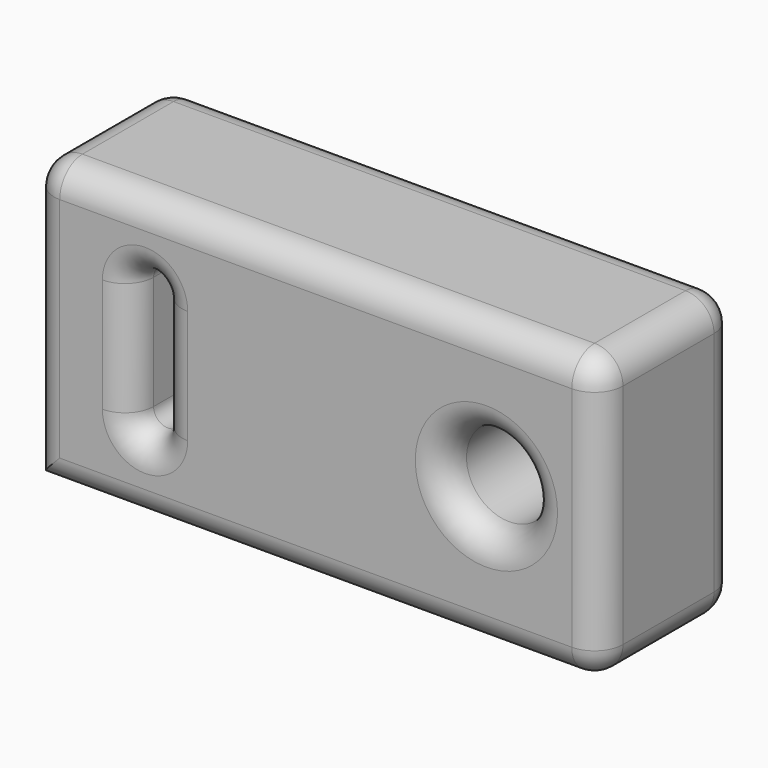
from build123d import *

# Parameters (mm, degrees)
F0_W         = 254
F0_H         = 127
F1_DEPTH     = 76.2
F2_R         = 19.05
F3_DEPTH     = 76.201
F5_DEPTH     = 76.201
F6_R         = 12.7
F7_T1_DEPTH  = 228.6
F7_T3_DEPTH  = 50.8
F7_T5_DEPTH  = 101.6
F7_T7_DEPTH  = 273.05
F7_T9_DEPTH  = 146.05
F7_T11_DEPTH = 50.8
F7_S15_W     = 12.7
F7_S15_H     = 12.7
F7_T16_DEPTH = 12.7
F7_S21_W     = 12.7
F7_S21_H     = 12.7
F7_T22_DEPTH = 12.7
F7_S27_W     = 12.7
F7_S27_H     = 12.7
F7_T28_DEPTH = 12.7
F7_S33_W     = 12.7
F7_S33_H     = 12.7
F7_T34_DEPTH = 12.7
F7_S39_W     = 12.7
F7_S39_H     = 12.7
F7_T40_DEPTH = 12.7
F7_S45_W     = 12.7
F7_S45_H     = 12.7
F7_T46_DEPTH = 12.7
F7_T50_ANGLE = 180
F7_T52_ANGLE = 180


# Not quite as in the source:
# - a fillet or chamfer that OpenCascade refuses, or shapes differently, is made with other operations: its cross-section is extruded or revolved along the edge and cut away or added


with BuildPart() as f1:
    # F0 (on Front) → F1 (new body)
    with BuildSketch(Plane.XZ):
        with Locations((127, 63.5)):
            Rectangle(F0_W, F0_H)
    extrude(amount=F1_DEPTH)

    # F2 (on face) → F3 (cut, through all)
    with BuildSketch(Plane.XZ.offset(76.2)):
        with Locations((203.2, 63.5)):
            Circle(F2_R)
    extrude(amount=-F3_DEPTH, mode=Mode.SUBTRACT)

    # F4 (on face) → F5 (cut, through all)
    with BuildSketch(Plane.XZ.offset(76.2)):
        with BuildLine():
            Line((57.15, 38.1), (57.15, 88.9))
            ThreePointArc((57.15, 88.9), (50.8, 95.25), (44.45, 88.9))
            Line((44.45, 88.9), (44.45, 38.1))
            ThreePointArc((44.45, 38.1), (50.8, 31.75), (57.15, 38.1))
        make_face()
    extrude(amount=-F5_DEPTH, mode=Mode.SUBTRACT)

    # F6
    f6_edges = [f1.edges().sort_by_distance(p)[0] for p in [
        (0, -76.2, 63.5),
        (127, -76.2, 127),
        (127, -76.2, 0),
        (254, -76.2, 63.5),
        (57.15, -76.2, 63.5),
        (50.8, -76.2, 95.25),
        (44.45, -76.2, 63.5),
        (50.8, -76.2, 31.75),
        (184.15, -76.2, 63.5),
    ]]
    fillet(f6_edges, radius=F6_R)

    # F7: fillet of radius 12.7 on 12 edges, made by hand

    # F7_s2 → F7_t1 (cut)
    with BuildSketch(Plane.YZ.offset(12.7)):
        with BuildLine():
            ThreePointArc((-12.7, 127), (-3.7197438789, 123.2802561211), (0, 114.3))
            Line((0, 114.3), (0, 127))
            Line((0, 127), (-12.7, 127))
        make_face()
    extrude(amount=F7_T1_DEPTH, mode=Mode.SUBTRACT)

    # F7_s4 → F7_t3 (cut)
    with BuildSketch(Plane.XZ.offset(12.7)):
        with BuildLine():
            ThreePointArc((0, 114.3), (3.7197438789, 123.2802561211), (12.7, 127))
            Line((12.7, 127), (0, 127))
            Line((0, 127), (0, 114.3))
        make_face()
        with BuildLine():
            ThreePointArc((241.3, 127), (250.2802561211, 123.2802561211), (254, 114.3))
            Line((254, 114.3), (254, 127))
            Line((254, 127), (241.3, 127))
        make_face()
        with BuildLine():
            ThreePointArc((241.3, 0), (250.2802561211, 3.7197438789), (254, 12.7))
            Line((254, 12.7), (254, 0))
            Line((254, 0), (241.3, 0))
        make_face()
    extrude(amount=F7_T3_DEPTH, mode=Mode.SUBTRACT)

    # F7_s6 → F7_t5 (cut)
    with BuildSketch(Plane.XY.offset(12.7)):
        with BuildLine():
            ThreePointArc((241.3, 0), (250.2802561211, -3.7197438789), (254, -12.7))
            Line((254, -12.7), (254, 0))
            Line((254, 0), (241.3, 0))
        make_face()
    extrude(amount=F7_T5_DEPTH, mode=Mode.SUBTRACT)

    # F7_s8 → F7_t7 (cut)
    with BuildSketch(Plane.YZ.offset(-31.75)):
        with BuildLine():
            ThreePointArc((0, 12.7), (-3.7197438789, 3.7197438789), (-12.7, 0))
            Line((-12.7, 0), (0, 0))
            Line((0, 0), (0, 12.7))
        make_face()
    extrude(amount=F7_T7_DEPTH, mode=Mode.SUBTRACT)

    # F7_s10 → F7_t9 (cut)
    with BuildSketch(Plane.XY.offset(-31.75)):
        with BuildLine():
            ThreePointArc((0, -12.7), (3.7197438789, -3.7197438789), (12.7, 0))
            Line((12.7, 0), (0, 0))
            Line((0, 0), (0, -12.7))
        make_face()
    extrude(amount=F7_T9_DEPTH, mode=Mode.SUBTRACT)

    # F7_s12 → F7_t11 (cut)
    with BuildSketch(Plane.XY.offset(38.1)):
        with BuildLine():
            ThreePointArc((31.75, 0), (40.7302561211, -3.7197438789), (44.45, -12.7))
            Line((44.45, -12.7), (44.45, 0))
            Line((44.45, 0), (31.75, 0))
        make_face()
        with BuildLine():
            ThreePointArc((69.85, 0), (60.8697438789, -3.7197438789), (57.15, -12.7))
            Line((57.15, -12.7), (57.15, 0))
            Line((57.15, 0), (69.85, 0))
        make_face()
    extrude(amount=F7_T11_DEPTH, mode=Mode.SUBTRACT)


with BuildPart() as f7_tool14:
    # F7_s15 → F7_t16 (new body)
    with BuildSketch(Plane.XY.offset(12.7)):
        with Locations((247.65, -69.85)):
            Rectangle(F7_S15_W, F7_S15_H)
    extrude(amount=-F7_T16_DEPTH)

    # F7_s17 → F7_t18 (revolve, cut)
    with BuildSketch(Plane(origin=(241.3, -63.5, 12.7), x_dir=(-0.7071067812, 0.7071067812, 0), z_dir=(-0.7071067812, -0.7071067812, 0))):
        with BuildLine():
            ThreePointArc((0, -12.7), (12.7, 0), (0, 12.7))
            Line((0, 12.7), (0, -12.7))
        make_face()
    revolve(axis=Axis((241.3, -63.5, 12.7), (0, 0, -1)), mode=Mode.SUBTRACT)


with BuildPart() as f1_1:
    add(f1.part)

    # F7_t13: cut F7_tool14
    add(f7_tool14.part, mode=Mode.SUBTRACT)


with BuildPart() as f7_tool20:
    # F7_s21 → F7_t22 (new body)
    with BuildSketch(Plane.XY.offset(114.3)):
        with Locations((247.65, -69.85)):
            Rectangle(F7_S21_W, F7_S21_H)
    extrude(amount=F7_T22_DEPTH)

    # F7_s23 → F7_t24 (revolve, cut)
    with BuildSketch(Plane(origin=(241.3, -63.5, 114.3), x_dir=(-0.7071067812, 0.7071067812, 0), z_dir=(0.7071067812, 0.7071067812, 0))):
        with BuildLine():
            ThreePointArc((0, -12.7), (12.7, 0), (0, 12.7))
            Line((0, 12.7), (0, -12.7))
        make_face()
    revolve(axis=Axis((241.3, -63.5, 114.3), (0, 0, 1)), mode=Mode.SUBTRACT)


with BuildPart() as f1_2:
    add(f1_1.part)

    # F7_t19: cut F7_tool20
    add(f7_tool20.part, mode=Mode.SUBTRACT)


with BuildPart() as f7_tool26:
    # F7_s27 → F7_t28 (new body)
    with BuildSketch(Plane.YZ.offset(12.7)):
        with Locations((-69.85, 120.65)):
            Rectangle(F7_S27_W, F7_S27_H)
    extrude(amount=-F7_T28_DEPTH)

    # F7_s29 → F7_t30 (revolve, cut)
    with BuildSketch(Plane(origin=(12.7, -63.5, 114.3), x_dir=(0, 0.7071067812, -0.7071067812), z_dir=(0, 0.7071067812, 0.7071067812))):
        with BuildLine():
            ThreePointArc((0, -12.7), (12.7, 0), (0, 12.7))
            Line((0, 12.7), (0, -12.7))
        make_face()
    revolve(axis=Axis((12.7, -63.5, 114.3), (-1, 0, 0)), mode=Mode.SUBTRACT)


with BuildPart() as f1_3:
    add(f1_2.part)

    # F7_t25: cut F7_tool26
    add(f7_tool26.part, mode=Mode.SUBTRACT)


with BuildPart() as f7_tool32:
    # F7_s33 → F7_t34 (new body)
    with BuildSketch(Plane.XY.offset(114.3)):
        with Locations((247.65, -6.35)):
            Rectangle(F7_S33_W, F7_S33_H)
    extrude(amount=F7_T34_DEPTH)

    # F7_s35 → F7_t36 (revolve, cut)
    with BuildSketch(Plane(origin=(241.3, -12.7, 114.3), x_dir=(-0.7071067812, -0.7071067812, 0), z_dir=(-0.7071067812, 0.7071067812, 0))):
        with BuildLine():
            ThreePointArc((0, -12.7), (12.7, 0), (0, 12.7))
            Line((0, 12.7), (0, -12.7))
        make_face()
    revolve(axis=Axis((241.3, -12.7, 114.3), (0, 0, 1)), mode=Mode.SUBTRACT)


with BuildPart() as f1_4:
    add(f1_3.part)

    # F7_t31: cut F7_tool32
    add(f7_tool32.part, mode=Mode.SUBTRACT)


with BuildPart() as f7_tool38:
    # F7_s39 → F7_t40 (new body)
    with BuildSketch(Plane.YZ.offset(12.7)):
        with Locations((-6.35, 120.65)):
            Rectangle(F7_S39_W, F7_S39_H)
    extrude(amount=-F7_T40_DEPTH)

    # F7_s41 → F7_t42 (revolve, cut)
    with BuildSketch(Plane(origin=(12.7, -12.7, 114.3), x_dir=(0, -0.7071067812, -0.7071067812), z_dir=(0, 0.7071067812, -0.7071067812))):
        with BuildLine():
            ThreePointArc((0, -12.7), (12.7, 0), (0, 12.7))
            Line((0, 12.7), (0, -12.7))
        make_face()
    revolve(axis=Axis((12.7, -12.7, 114.3), (-1, 0, 0)), mode=Mode.SUBTRACT)


with BuildPart() as f1_5:
    add(f1_4.part)

    # F7_t37: cut F7_tool38
    add(f7_tool38.part, mode=Mode.SUBTRACT)


with BuildPart() as f7_tool44:
    # F7_s45 → F7_t46 (new body)
    with BuildSketch(Plane.XZ.offset(12.7)):
        with Locations((247.65, 6.35)):
            Rectangle(F7_S45_W, F7_S45_H)
    extrude(amount=-F7_T46_DEPTH)

    # F7_s47 → F7_t48 (revolve, cut)
    with BuildSketch(Plane(origin=(241.3, -12.7, 12.7), x_dir=(-0.7071067812, 0, 0.7071067812), z_dir=(-0.7071067812, 0, -0.7071067812))):
        with BuildLine():
            ThreePointArc((0, -12.7), (12.7, 0), (0, 12.7))
            Line((0, 12.7), (0, -12.7))
        make_face()
    revolve(axis=Axis((241.3, -12.7, 12.7), (0, 1, 0)), mode=Mode.SUBTRACT)


with BuildPart() as f1_6:
    add(f1_5.part)

    # F7_t43: cut F7_tool44
    add(f7_tool44.part, mode=Mode.SUBTRACT)

    # F7_s49 → F7_t50 (revolve, cut)
    with BuildSketch(Plane.XY.offset(38.1)):
        with BuildLine():
            ThreePointArc((31.75, 0), (40.7302561211, -3.7197438789), (44.45, -12.7))
            Line((44.45, -12.7), (44.45, 0))
            Line((44.45, 0), (31.75, 0))
        make_face()
    revolve(axis=Axis((50.8, 0, 38.1), (0, -1, 0)), revolution_arc=F7_T50_ANGLE, mode=Mode.SUBTRACT)

    # F7_s51 → F7_t52 (revolve, cut)
    with BuildSketch(Plane.XY.offset(88.9)):
        with BuildLine():
            ThreePointArc((69.85, 0), (60.8697438789, -3.7197438789), (57.15, -12.7))
            Line((57.15, -12.7), (57.15, 0))
            Line((57.15, 0), (69.85, 0))
        make_face()
    revolve(axis=Axis((50.8, 0, 88.9), (0, -1, 0)), revolution_arc=F7_T52_ANGLE, mode=Mode.SUBTRACT)

    # F7_s53 → F7_t54 (revolve, cut)
    with BuildSketch(Plane.XY.offset(63.5)):
        with BuildLine():
            ThreePointArc((234.95, 0), (225.9697438789, -3.7197438789), (222.25, -12.7))
            Line((222.25, -12.7), (222.25, 0))
            Line((222.25, 0), (234.95, 0))
        make_face()
    revolve(axis=Axis((203.2, 0, 63.5), (0, -1, 0)), mode=Mode.SUBTRACT)


solid = f1_6.part
